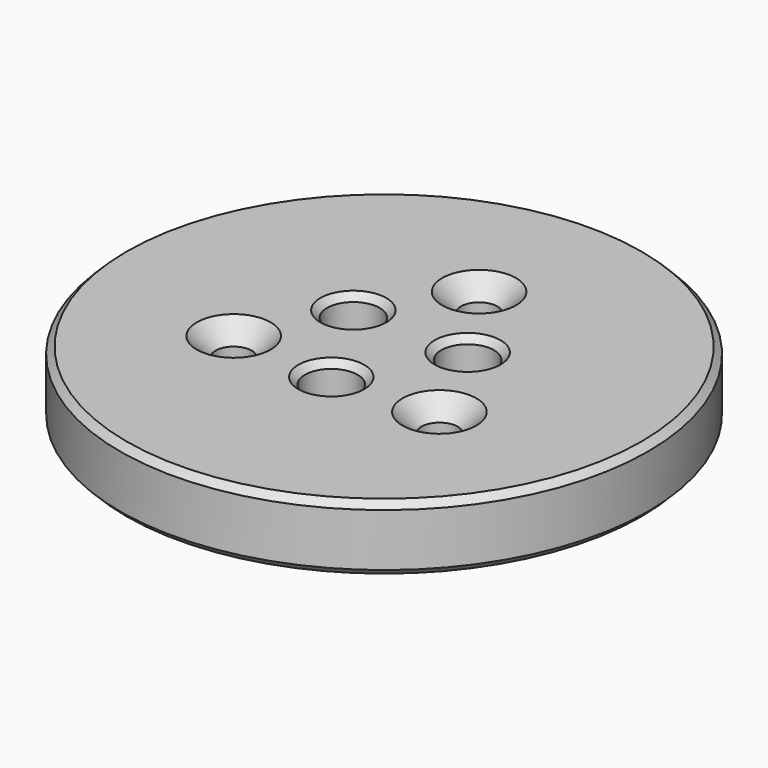
from build123d import *

# Parameters (mm, degrees)
F0_R            = 40
F2_DEPTH        = 10
F3_D            = 5.5
F3_CSINK_D      = 11.2
F3_CSINK_ANGLE  = 90
F3_COPIES_COUNT = 3
F4_R            = 4
F5_DEPTH        = 8
F5_COPIES_COUNT = 3
F6_SIZE         = 1


# Not quite as in the source:
# - a pattern or mirror of a feature is missing from the dataset's text; its kind, count and spacing are read off the source's solid
# - a feature names something its author has since deleted; it is built from what else it names


with BuildPart() as f2:
    # F0 (on Top) → F2 (new body)
    with BuildSketch(Plane.XY):
        Circle(F0_R)
    extrude(amount=-F2_DEPTH)

    # F3 (through all)
    with Locations(Plane.XY):
        with Locations((0, 18)):
            f3 = CounterSinkHole(F3_D / 2, F3_CSINK_D / 2, counter_sink_angle=F3_CSINK_ANGLE)

    # F3_copies: F3 ×3 about axis
    f3_copies_axis = Axis((0, 0, 0), (0, 0, 1))
    for i in range(1, F3_COPIES_COUNT):
        add(f3.rotate(f3_copies_axis, i * 360 / F3_COPIES_COUNT), mode=Mode.SUBTRACT)

    # F4 (on face) → F5 (cut)
    with BuildSketch(Plane.XY):
        with Locations((0, -10)):
            Circle(F4_R)
    f5 = extrude(amount=-F5_DEPTH, mode=Mode.SUBTRACT)

    # F5_copies: F5 ×3 about axis
    f5_copies_axis = Axis((0, 0, 0), (0, 0, 1))
    for i in range(1, F5_COPIES_COUNT):
        add(f5.rotate(f5_copies_axis, i * 360 / F5_COPIES_COUNT), mode=Mode.SUBTRACT)

    # F6
    f6_edges = [f2.edges().sort_by_distance(p)[0] for p in [
        (-40, 0, -10),
        (-40, 0, 0),
        (-4, -10, 0),
        (-6.660254, 8.464102, 0),
        (10.660254, 1.535898, 0),
    ]]
    chamfer(f6_edges, length=F6_SIZE)


solid = f2.part
